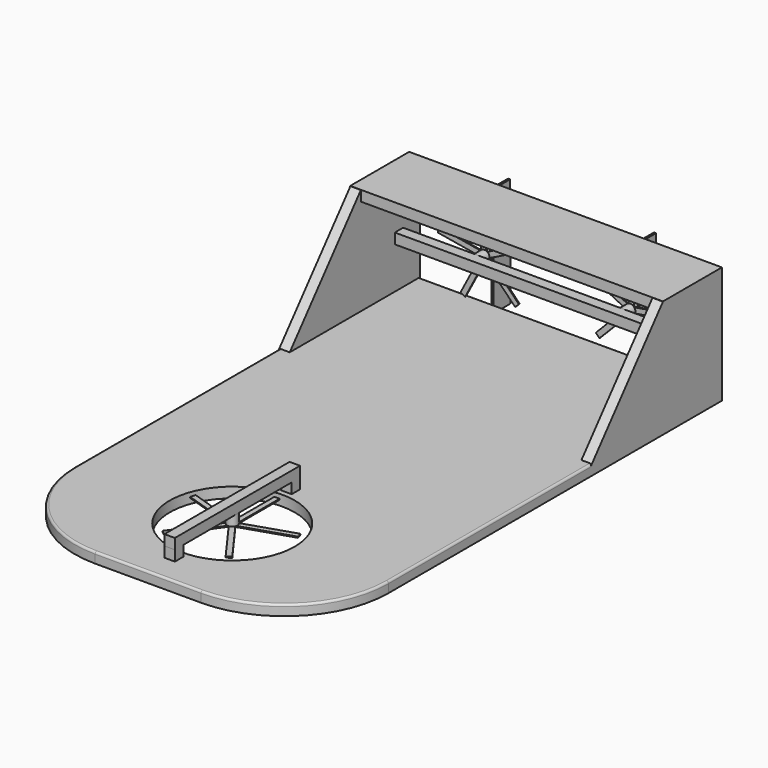
from build123d import *

# Parameters (mm, degrees)
F0_R      = 152.4
F1_DEPTH  = 25.4
F2_R      = 5.08
F3_W      = 25.4
F3_H      = 25.4
F3_H_2    = 25.8285974579
F4_DEPTH  = 25.4
F5_W      = 25.4
F5_H      = 381.3520879745
F6_DEPTH  = 25.4
F8_DEPTH  = 25.4
F11_DEPTH = 25.4
F12_W     = 25.4
F12_H     = 25.4
F13_DEPTH = 711.2
F14_R     = 12.7
F14_R_2   = 11.43
F15_DEPTH = 25.4
F17_DEPTH = 2.54
F19_DEPTH = 50.8
F20_R     = 12.7
F20_R_2   = 11.43
F21_DEPTH = 25.4
F23_DEPTH = 2.54


# Not quite as in the source:
# - the program builds the solid bodies; features that only make, move or delete a surface that nothing else refers to are left out


with BuildPart() as f1:
    # F0 (on Top) → F1 (new body)
    with BuildSketch(Plane.XY):
        with BuildLine():
            Line((381, 635), (-381, 635))
            Line((-381, 635), (-381, -385))
            ThreePointArc((-381, -385), (-307.7766952966, -561.7766952966), (-131, -635))
            Line((-131, -635), (127, -635))
            ThreePointArc((127, -635), (306.6051224214, -560.6051224214), (381, -381))
            Line((381, -381), (381, 635))
        make_face()
        with Locations((0, -381)):
            Circle(F0_R, mode=Mode.SUBTRACT)
    extrude(amount=-F1_DEPTH)

    # F2
    f2_edges = [f1.edges().sort_by_distance(p)[0] for p in [
        (-381, 125, 0),
        (-307.776695, -561.776695, 0),
        (-2, -635, 0),
        (306.605122, -560.605122, 0),
        (381, 127, 0),
        (0, 635, 0),
    ]]
    fillet(f2_edges, radius=F2_R)

    # F3 (on face) → F4 (join)
    with BuildSketch(Plane.XY):
        with Locations((0, -203.2)):
            Rectangle(F3_W, F3_H)
        with Locations((0, -558.8)):
            Rectangle(F3_W, F3_H_2)
    extrude(amount=F4_DEPTH)

    # F5 (on face) → F6 (join)
    with BuildSketch(Plane.XY.offset(25.4)):
        with Locations((0, -381.1760439873)):
            Rectangle(F5_W, F5_H)
    extrude(amount=F6_DEPTH)

    # F9: F8 across plane


with BuildPart() as f8:
    # F7 (on face) → F8 (new body)
    with BuildSketch(Plane.YZ.offset(381)):
        Polygon((234.4024777412, -5.08), (635, -5.08), (635, 260.7663869858), (455.7277560234, 260.7663869858), align=None)
    extrude(amount=-F8_DEPTH)


with BuildPart() as f1_1:
    add(f1.part)
    add(f8.part.mirror(Plane.YZ))


    add(f8.part)  # F11 merges F8
    # F10 (on face) → F11 (join)
    with BuildSketch(Plane.XY.offset(260.7663869858)):
        Polygon((355.6, 455.7277560234), (355.6, 635), (-381.5401494503, 635), (-381.5401494503, 455.294251442), (381, 455.294251442), (381, 455.7277560234), align=None)
    extrude(amount=-F11_DEPTH)

    # F12 (on face) → F13 (join, through all)
    with BuildSketch(Plane(origin=(355.6, 0, 0), x_dir=(0, -1, 0), z_dir=(-1, 0, 0))):
        with Locations((-571.5, 114.3)):
            Rectangle(F12_W, F12_H)
    extrude(amount=F13_DEPTH)

    # F18 (on face) → F19 (join)
    with BuildSketch(Plane(origin=(0, 635, 0), x_dir=(-1, 0, 0), z_dir=(0, 1, 0))):
        Polygon((-180.3399947906, -18.6284687443), (-175.2600052094, -18.6387572841), (-174.7198557591, 248.0612427159), (-179.7998453403, 248.0715312557), align=None)
        Polygon((180.8801442409, 248.0612427159), (175.8001546597, 248.0715312557), (175.2600052094, -18.6284687443), (180.3399947906, -18.6387572841), align=None)
    extrude(amount=F19_DEPTH)

    # F20 (on face) → F21 (join)
    with BuildSketch(Plane(origin=(0, 0, 25.4), x_dir=(1, 0, 0), z_dir=(0, 0, -1))):
        with Locations((0, 381)):
            Circle(F20_R)
        with Locations((0, 381)):
            Circle(F20_R_2, mode=Mode.SUBTRACT)
    extrude(amount=F21_DEPTH)


with BuildPart() as f15:
    # F14 (on face) → F15 (new body)
    with BuildSketch(Plane(origin=(0, 584.2, 0), x_dir=(-1, 0, 0), z_dir=(0, 1, 0))):
        with Locations((-177.8, 114.3)):
            Circle(F14_R)
        with Locations((-177.8, 114.3)):
            Circle(F14_R_2, mode=Mode.SUBTRACT)
    extrude(amount=F15_DEPTH)


with BuildPart() as f15b:
    # F14 (on face) → F15, piece 2 (new body)
    with BuildSketch(Plane(origin=(0, 584.2, 0), x_dir=(-1, 0, 0), z_dir=(0, 1, 0))):
        with Locations((177.8, 114.3)):
            Circle(F14_R)
        with Locations((177.8, 114.3)):
            Circle(F14_R_2, mode=Mode.SUBTRACT)
    extrude(amount=F15_DEPTH)


with BuildPart() as f17:
    # F16 (on face) → F17 (new body)
    with BuildSketch(Plane(origin=(0, 609.6, 0), x_dir=(-1, 0, 0), z_dir=(0, 1, 0))):
        Polygon((-176.2287217864, 103.6116089142), (-173.1315717637, 109.5266083861), (-167.1491895745, 112.4914773008), (-171.8176097634, 117.2648706101), (-172.7887111674, 123.8706576668), (-178.771098065, 120.9057864186), (-185.3536605461, 122.0235143615), (-184.382560212, 115.4177345825), (-187.4797086447, 109.5027381472), (-180.8971505009, 108.3850109408), align=None)
        Polygon((-167.1491895745, 112.4914773008), (-173.1315717637, 109.5266083861), (-176.2287217864, 103.6116089142), (-102.8278704973, 28.560281428), (-93.7483348442, 37.4401462961), align=None)
        Polygon((-171.8176097634, 117.2648706101), (-167.1491895745, 112.4914773008), (-73.089019826, 159.1077021724), (-78.7285420374, 170.4868822318), (-172.7887111674, 123.8706576668), align=None)
        Polygon((-224.9246668441, 10.6111125903), (-176.2287217864, 103.6116089142), (-180.8971505009, 108.3850109408), (-187.4797086447, 109.5027381472), (-236.1756559324, 16.5022375643), align=None)
        Polygon((-178.771098065, 120.9057864186), (-172.7887111674, 123.8706576668), (-188.0571847598, 227.7324014723), (-200.6221340373, 225.8852574787), (-185.3536605461, 122.0235143615), align=None)
        Polygon((-290.976313686, 127.0766005719), (-187.4797086447, 109.5027381472), (-184.382560212, 115.4177345825), (-185.3536605461, 122.0235143615), (-288.8502689845, 139.597377363), align=None)
    extrude(amount=F17_DEPTH)


with BuildPart() as f17b:
    # F16 (on face) → F17, piece 2 (new body)
    with BuildSketch(Plane(origin=(0, 609.6, 0), x_dir=(-1, 0, 0), z_dir=(0, 1, 0))):
        Polygon((172.7887111674, 123.8706576668), (178.771098065, 120.9057864186), (185.3536605461, 122.0235143615), (200.6221340373, 225.8852574787), (188.0571847598, 227.7324014723), align=None)
        Polygon((185.3536605461, 122.0235143615), (178.771098065, 120.9057864186), (172.7887111674, 123.8706576668), (171.8176097634, 117.2648706101), (167.1491895745, 112.4914773008), (173.1315717637, 109.5266083861), (176.2287217864, 103.6116089142), (180.8971505009, 108.3850109408), (187.4797086447, 109.5027381472), (184.382560212, 115.4177345825), align=None)
        Polygon((288.8502689845, 139.597377363), (185.3536605461, 122.0235143615), (184.382560212, 115.4177345825), (187.4797086447, 109.5027381472), (290.976313686, 127.0766005719), align=None)
        Polygon((171.8176097634, 117.2648706101), (172.7887111674, 123.8706576668), (78.7285420374, 170.4868822318), (73.089019826, 159.1077021724), (167.1491895745, 112.4914773008), align=None)
        Polygon((236.1756559324, 16.5022375643), (187.4797086447, 109.5027381472), (180.8971505009, 108.3850109408), (176.2287217864, 103.6116089142), (224.9246668441, 10.6111125903), align=None)
        Polygon((173.1315717637, 109.5266083861), (167.1491895745, 112.4914773008), (93.7483348442, 37.4401462961), (102.8278704973, 28.560281428), (176.2287217864, 103.6116089142), align=None)
    extrude(amount=F17_DEPTH)


with BuildPart() as f23:
    # F22 (on face) → F23 (new body)
    with BuildSketch(Plane(origin=(0, 0, 0), x_dir=(1, 0, 0), z_dir=(0, 0, -1))):
        Polygon((6.3499999233, 372.2599748299), (2.16544e-05, 374.3232078401), (-6.35, 372.2599607331), (-6.35, 244.6820527577), (6.3499999233, 244.6820527577), align=None)
        Polygon((-6.35, 372.2599607331), (2.16544e-05, 374.3232078401), (6.3499999233, 372.2599748299), (6.3499999233, 378.9367598233), (10.2745163884, 384.3383933324), (3.9245149228, 386.4016338797), (5.85e-08, 391.8032651855), (-3.9245156754, 386.4016326828), (-10.2745080358, 384.338395094), (-6.35, 378.9367731868), align=None)
        Polygon((-127.6838099629, 332.8362160572), (-6.35, 372.2599607331), (-6.35, 378.9367731868), (-10.2745080358, 384.338395094), (-131.6083299271, 344.9146465423), align=None)
        Polygon((6.3499999233, 378.9367598233), (6.3499999233, 372.2599748299), (127.6838140985, 332.8362287853), (131.608330207, 344.9146474037), (10.2745163884, 384.3383933324), align=None)
        Polygon((-85.2629306216, 487.5511041858), (-10.2745080358, 384.338395094), (-3.9245156754, 386.4016326828), (5.85e-08, 391.8032651855), (-74.9884210975, 495.0159723094), align=None)
        Polygon((3.9245149228, 386.4016338797), (10.2745163884, 384.3383933324), (85.2629369261, 487.5510996053), (74.9884211741, 495.0159722538), (5.85e-08, 391.8032651855), align=None)
    extrude(amount=F23_DEPTH)


solid = Compound([f1_1.part, f15.part, f15b.part, f17.part, f17b.part, f23.part])
